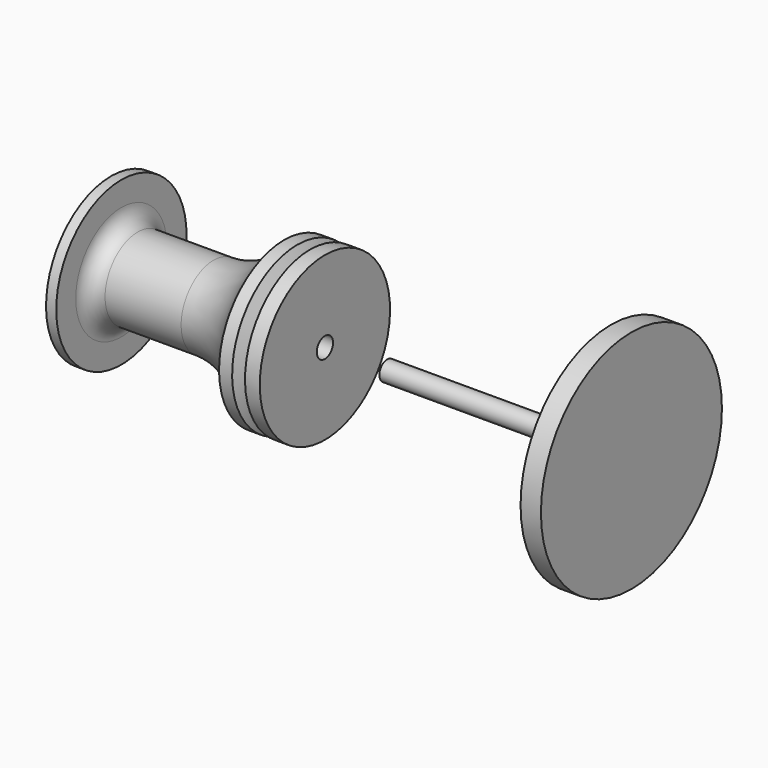
from build123d import *

# Parameters (mm, degrees)
F3_R     = 3.175
F4_DEPTH = 66.676
F5_R     = 5.08


# Not quite as in the source:
# - a fillet or chamfer that OpenCascade refuses, or shapes differently, is made with other operations: its cross-section is extruded or revolved along the edge and cut away or added


with BuildPart() as f1:
    # F0 (on Front) → F1 (revolve)
    with BuildSketch(Plane.XZ):
        Polygon((-70.8155093496, 25.4), (-70.8155093496, 0), (-4.1405093496, 0), (-4.1405093496, 25.4), (-8.7504833937, 25.4), (-10.7583906502, 20.8912156522), (-12.7662979066, 25.4), (-16.8405093496, 25.4), (-16.8405093496, 12.7), (-67.6405093496, 12.7), (-67.6405093496, 25.4), align=None)
    revolve(axis=Axis((-2.6019513607, 0, 0), (1, 0, 0)))

    # F2: fillet of radius 25.4 on 1 edges, made by hand

    # F2_s1 → F2_t2 (revolve)
    with BuildSketch(Plane.XZ):
        with BuildLine():
            ThreePointArc((-38.8375546057, 12.7), (-26.1375546057, 16.1029547439), (-16.8405093496, 25.4))
            Line((-16.8405093496, 25.4), (-16.4005684445, 25.146))
            ThreePointArc((-16.4005684445, 25.146), (-16.3325093496, 19.05), (-16.3325093496, 12.7))
            Line((-16.3325093496, 12.7), (-16.8405093496, 12.192))
            Line((-16.8405093496, 12.192), (-38.8375546057, 12.192))
            Line((-38.8375546057, 12.192), (-38.8375546057, 12.7))
        make_face()
    revolve(axis=Axis((-16.8405093496, 0, 0), (1, 0, 0)))

    # F3 (on face) → F4 (cut, through all)
    with BuildSketch(Plane.YZ.offset(-4.1405093496)):
        Circle(F3_R)
    extrude(amount=-F4_DEPTH, mode=Mode.SUBTRACT)

    # F5
    f5_edges = [f1.edges().sort_by_distance(p)[0] for p in [
        (-67.640509, 0, -12.7),
    ]]
    fillet(f5_edges, radius=F5_R)


with BuildPart() as f7:
    # F6 (on Front) → F7 (revolve)
    with BuildSketch(Plane.XZ):
        Polygon((15.2796903457, 3.048), (15.2796903457, 0), (91.4796903457, 0), (91.4796903457, 35.2887990795), (85.1296903457, 35.2887990795), (85.1296903457, 3.048), align=None)
    revolve(axis=Axis((53.1151062219, 0, 0), (1, 0, 0)))


solid = Compound([f1.part, f7.part])
